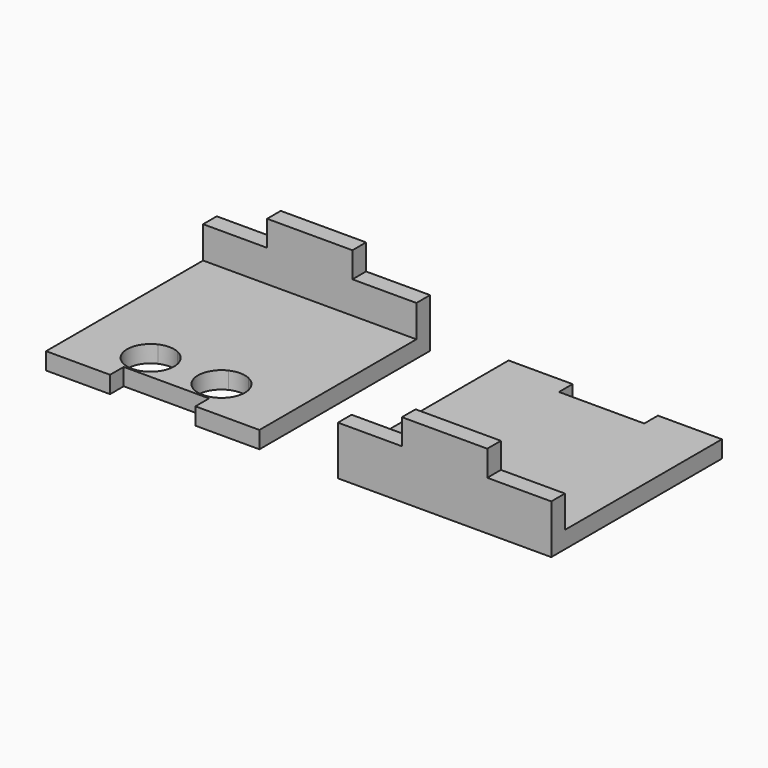
from build123d import *

# Parameters (mm, degrees)
F0_W      = 25
F0_H      = 2
F0_H_2    = 21
F1_DEPTH  = 2
F2_W      = 25
F2_H      = 2
F4_DEPTH  = 3.75
F3_W      = 25
F3_H      = 2
F5_W      = 10
F5_H      = 2
F7_DEPTH  = 2.001
F8_W      = 10
F8_H      = 2
F9_DEPTH  = 3
F10_W     = 10
F10_H     = 2
F11_DEPTH = 3
F13_DEPTH = 2
F15_DEPTH = 2.001
F17_DEPTH = 2.001


# Not quite as in the source:
# - a feature names something its author has since deleted; it is built from what else it names


with BuildPart() as f1:
    # F0 (on Top) → F1 (new body)
    with BuildSketch(Plane.XY):
        with Locations((-34.2000119388, 11.4999952018)):
            Rectangle(F0_W, F0_H)
        with Locations((-34.2000119388, -4.7982e-06)):
            Rectangle(F0_W, F0_H_2)
        with Locations((-34.2000119388, -11.5000047982)):
            Rectangle(F0_W, F0_H)
    extrude(amount=F1_DEPTH)

    # F2 (on face) → F4 (join)
    with BuildSketch(Plane.XY.offset(2)):
        with Locations((-34.2000119388, 11.4999952018)):
            Rectangle(F2_W, F2_H)
    extrude(amount=F4_DEPTH)

    # F5 (on face) → F7 (cut, through all)
    with BuildSketch(Plane.XY.offset(2)):
        with Locations((-34.2000119388, -11.5000047982)):
            Rectangle(F5_W, F5_H)
    extrude(amount=-F7_DEPTH, mode=Mode.SUBTRACT)

    # F8 (on face) → F9 (join)
    with BuildSketch(Plane.XY.offset(5.75)):
        with Locations((-34.2000119388, 11.4999952018)):
            Rectangle(F8_W, F8_H)
    extrude(amount=F9_DEPTH)

    # F16 (on face) → F17 (cut, through all)
    with BuildSketch(Plane.XY.offset(2)):
        with BuildLine():
            ThreePointArc((-39.5456558625, -5.0601771846), (-41.1500119388, -7.5601771846), (-39.5456558625, -10.0601771846))
            Line((-39.5456558625, -10.0601771846), (-37.2543680151, -10.0601771846))
            ThreePointArc((-37.2543680151, -10.0601771846), (-36.0855983208, -9.045434605), (-35.6500119388, -7.5601771846))
            ThreePointArc((-35.6500119388, -7.5601771846), (-36.0855983208, -6.0749197642), (-37.2543680151, -5.0601771846))
            Line((-37.2543680151, -5.0601771846), (-39.5456558625, -5.0601771846))
        make_face()
        with BuildLine():
            ThreePointArc((-37.2543680151, -5.0601771846), (-38.4000119388, -4.8101771846), (-39.5456558625, -5.0601771846))
            Line((-39.5456558625, -5.0601771846), (-37.2543680151, -5.0601771846))
        make_face()
        with BuildLine():
            Line((-37.2543680151, -10.0601771846), (-39.5456558625, -10.0601771846))
            ThreePointArc((-39.5456558625, -10.0601771846), (-38.4000119388, -10.3101771846), (-37.2543680151, -10.0601771846))
        make_face()
        with BuildLine():
            Line((-28.9543680151, -10.0601771846), (-31.2456558625, -10.0601771846))
            ThreePointArc((-31.2456558625, -10.0601771846), (-30.1000119388, -10.3101771846), (-28.9543680151, -10.0601771846))
        make_face()
        with BuildLine():
            ThreePointArc((-31.2456558625, -5.0601771846), (-32.8500119388, -7.5601771846), (-31.2456558625, -10.0601771846))
            Line((-31.2456558625, -10.0601771846), (-28.9543680151, -10.0601771846))
            ThreePointArc((-28.9543680151, -10.0601771846), (-27.7855983208, -9.045434605), (-27.3500119388, -7.5601771846))
            ThreePointArc((-27.3500119388, -7.5601771846), (-27.7855983208, -6.0749197642), (-28.9543680151, -5.0601771846))
            Line((-28.9543680151, -5.0601771846), (-31.2456558625, -5.0601771846))
        make_face()
        with BuildLine():
            ThreePointArc((-28.9543680151, -5.0601771846), (-30.1000119388, -4.8101771846), (-31.2456558625, -5.0601771846))
            Line((-31.2456558625, -5.0601771846), (-28.9543680151, -5.0601771846))
        make_face()
    extrude(amount=-F17_DEPTH, mode=Mode.SUBTRACT)


with BuildPart() as f1b:
    # F0 (on Top) → F1, piece 2 (new body)
    with BuildSketch(Plane.XY):
        with Locations((0, -11.5)):
            Rectangle(F0_W, F0_H)
        Rectangle(F0_W, F0_H_2)
        with Locations((0, 11.5)):
            Rectangle(F0_W, F0_H)
    extrude(amount=F1_DEPTH)

    # F3 (on face) → F4, piece 2 (join)
    with BuildSketch(Plane.XY.offset(2)):
        with Locations((0, -11.5)):
            Rectangle(F3_W, F3_H)
    extrude(amount=F4_DEPTH)

    # F10 (on face) → F11 (join)
    with BuildSketch(Plane.XY.offset(5.75)):
        with Locations((0, -11.5)):
            Rectangle(F10_W, F10_H)
    extrude(amount=F11_DEPTH)

    # F12 (on face) → F13 (cut)
    with BuildSketch(Plane(origin=(0, 12.5, 0), x_dir=(-1, 0, 0), z_dir=(0, 1, 0))):
        Polygon((-5, 2), (-5, 1), (0, 1), (5, 1), (5, 2), align=None)
        Polygon((0, 1), (-5, 1), (-5, 0), (5, 0), (5, 1), align=None)
    extrude(amount=-F13_DEPTH, mode=Mode.SUBTRACT)

    # F14 (on face) → F15 (cut, through all)
    with BuildSketch(Plane.XY.offset(2)):
        with BuildLine():
            Line((-4.2448268481, -10.4756355286), (-4.1551731519, -10.4756355286))
            ThreePointArc((-4.1551731519, -10.4756355286), (-2.4164547777, -9.7278840301), (-1.7, -7.9760374501))
            ThreePointArc((-1.7, -7.9760374501), (-5.95184658, -6.1924922278), (-4.2448268481, -10.4756355286))
        make_face()
        with BuildLine():
            Line((4.0551731519, -10.4756355286), (4.1448268481, -10.4756355286))
            ThreePointArc((4.1448268481, -10.4756355286), (5.8835452223, -9.7278840301), (6.6, -7.9760374501))
            ThreePointArc((6.6, -7.9760374501), (2.34815342, -6.1924922278), (4.0551731519, -10.4756355286))
        make_face()
    extrude(amount=-F15_DEPTH, mode=Mode.SUBTRACT)


solid = Compound([f1.part, f1b.part])
